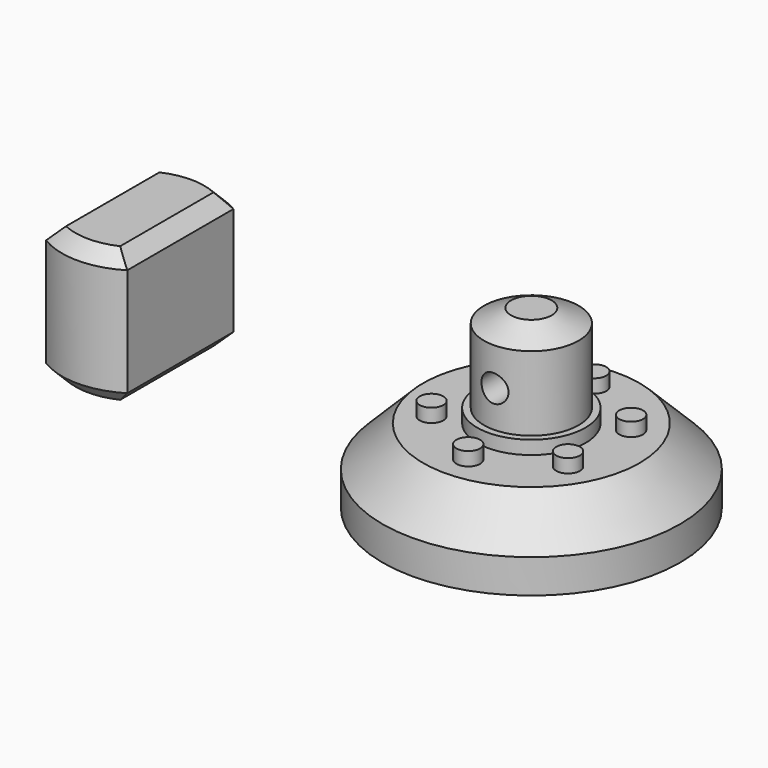
from build123d import *

# Parameters (mm, degrees)
F0_W        = 6
F0_H        = 9.8107084352
F1_DEPTH    = 10
F2_SIZE     = 1
F3_R        = 11
F4_DEPTH    = 5.5
F5_SIZE     = 3
F6_R        = 0.875
F7_DEPTH    = 6.5
F8_COUNT    = 6
F9_R        = 4
F10_DEPTH   = 6.5
F11_R       = 3.5
F12_DEPTH   = 13
F13_SIZE2   = 1
F13_SIZE    = 2
F15_DEPTH   = 6
F16_C1_SIZE = 3
F16_C2_SIZE = 3
F16_C3_SIZE = 3
F16_C4_SIZE = 3
F18_R       = 1
F19_DEPTH   = 4


with BuildPart() as f1:
    # F0 (on Top) → F1 (new body)
    with BuildSketch(Plane.XY):
        with BuildLine():
            Line((-31.9442992674, 4.9053542176), (-25.9442992674, 4.9053542176))
            ThreePointArc((-25.9442992674, 4.9053542176), (-28.9442992674, 5.75), (-31.9442992674, 4.9053542176))
        make_face()
        with Locations((-28.9442992674, 0)):
            Rectangle(F0_W, F0_H)
        with BuildLine():
            ThreePointArc((-31.9442992674, -4.9053542176), (-28.9442992674, -5.75), (-25.9442992674, -4.9053542176))
            Line((-25.9442992674, -4.9053542176), (-31.9442992674, -4.9053542176))
        make_face()
    extrude(amount=F1_DEPTH)

    # F2
    f2_edges = [f1.edges().sort_by_distance(p)[0] for p in [
        (-28.944299, 5.75, 10),
        (-31.944299, 0, 10),
        (-28.944299, -5.75, 10),
        (-25.944299, 0, 10),
        (-28.944299, 5.75, 0),
        (-31.944299, 0, 0),
        (-28.944299, -5.75, 0),
        (-25.944299, 0, 0),
    ]]
    chamfer(f2_edges, length=F2_SIZE)


with BuildPart() as f4:
    # F3 (on Top) → F4 (new body)
    with BuildSketch(Plane.XY):
        Circle(F3_R)
    extrude(amount=F4_DEPTH)

    # F5
    f5_edges = [f4.edges().sort_by_distance(p)[0] for p in [
        (-11, 0, 5.5),
    ]]
    chamfer(f5_edges, length=F5_SIZE)

    # F6 (on Top) → F7 (join)
    with BuildSketch(Plane.XY):
        with Locations((0, -5.8274352923)):
            Circle(F6_R)
    extrude(amount=F7_DEPTH)

    # F8: F4 ×6 about axis
    f8_axis = Axis((0, 0, 5.5), (0, 0, 1))


with BuildPart() as f4_1:
    add(f4.part)
    for i in range(1, F8_COUNT):
        add(f4.part.rotate(f8_axis, i * 360 / F8_COUNT))

    # F9 (on Top) → F10 (join)
    with BuildSketch(Plane.XY):
        Circle(F9_R)
    extrude(amount=F10_DEPTH)

    # F11 (on Top) → F12 (join)
    with BuildSketch(Plane.XY):
        Circle(F11_R)
    extrude(amount=F12_DEPTH)

    # F13
    f13_edges = [f4_1.edges().sort_by_distance(p)[0] for p in [
        (-3.5, 0, 13),
    ]]
    f13_side = f4_1.faces().sort_by_distance((0, 0, 13))[0]
    chamfer(f13_edges, length=F13_SIZE, length2=F13_SIZE2, reference=f13_side)


with BuildPart() as f15:
    # F14 (on Top) → F15 (new body)
    with BuildSketch(Plane.XY):
        with BuildLine():
            Line((-3.2844228611, 5.110756855), (-3.2844228611, -4.976363646))
            ThreePointArc((-3.2844228611, -4.976363646), (-0.0344228611, -5.9328033955), (3.2155771389, -4.976363646))
            Line((3.2155771389, -4.976363646), (3.2155771389, 5.110756855))
            ThreePointArc((3.2155771389, 5.110756855), (-0.0344228611, 6.0671966045), (-3.2844228611, 5.110756855))
        make_face()
    extrude(amount=F15_DEPTH)

    # F16: chamfer of 3 on 4 edges, made by hand

    # F16_c1
    f16_c1_edges = [f15.edges().sort_by_distance(p)[0] for p in [
        (3.2155771389, 0.0671966045, 6),
    ]]
    chamfer(f16_c1_edges, length=F16_C1_SIZE)

    # F16_c2
    f16_c2_edges = [f15.edges().sort_by_distance(p)[0] for p in [
        (-3.2844228611, 0.0671966045, 6),
    ]]
    chamfer(f16_c2_edges, length=F16_C2_SIZE)

    # F16_c3
    f16_c3_edges = [f15.edges().sort_by_distance(p)[0] for p in [
        (-0.0344228611, -5.9328033955, 6),
    ]]
    chamfer(f16_c3_edges, length=F16_C3_SIZE)

    # F16_c4
    f16_c4_edges = [f15.edges().sort_by_distance(p)[0] for p in [
        (-0.0344228611, 6.0671966045, 6),
    ]]
    chamfer(f16_c4_edges, length=F16_C4_SIZE)


with BuildPart() as f4_2:
    add(f4_1.part)

    # F17: cut F15
    add(f15.part, mode=Mode.SUBTRACT)

    # F18 (on Front) → F19 (cut)
    with BuildSketch(Plane.XZ):
        with Locations((0, 9.1908816248)):
            Circle(F18_R)
    extrude(amount=F19_DEPTH, mode=Mode.SUBTRACT)


solid = Compound([f1.part, f4_2.part])
